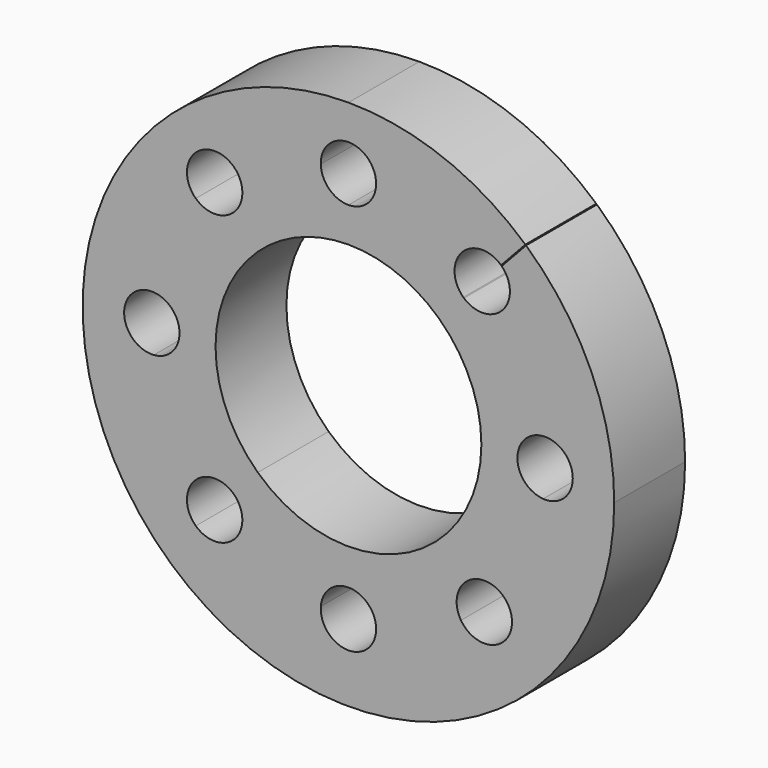
from build123d import *

# Parameters (mm, degrees)
F1_DEPTH = 25.4


# Not quite as in the source:
# - ends of sketch curves that miss each other by under 0.0002 mm in the source are joined


with BuildPart() as f1:
    # F0 (on Front) → F1 (new body)
    with BuildSketch(Plane.XZ):
        with BuildLine():
            ThreePointArc((7.9345325801, 55.8050164826), (5.535399088, 50.3331676174), (0, 48.0845394904))
            ThreePointArc((0, 48.0845394904), (-5.53484385, 50.3326274112), (-7.9344900677, 55.8034677281))
            ThreePointArc((-7.9344900677, 55.8034677281), (-20.6052011609, 52.4624086595), (-32.1621766165, 46.2861708383))
            ThreePointArc((-32.1621766165, 46.2861708383), (-30.8592654267, 43.9476457313), (-30.4078463876, 41.3089911317))
            ThreePointArc((-30.4078463876, 41.3089911317), (-31.0665806395, 38.1430038554), (-32.9334464969, 35.5025080461))
            ThreePointArc((-32.9334464969, 35.5025080461), (-38.3527879746, 33.37149462), (-43.7681241803, 35.5126658077))
            ThreePointArc((-43.7681241803, 35.5126658077), (-51.6631141521, 22.5336801806), (-55.8055284532, 7.9177526246))
            ThreePointArc((-55.8055284532, 7.9177526246), (-50.5579583584, 5.4112130729), (-48.4275815127, 0))
            ThreePointArc((-48.4275815127, 0), (-50.5584477046, -5.4117381745), (-55.8069604277, -7.917853693))
            ThreePointArc((-55.8069604277, -7.917853693), (-51.6665413057, -22.5360169357), (-43.772503534, -35.5174627239))
            ThreePointArc((-43.772503534, -35.5174627239), (-38.3573927277, -33.3769597298), (-32.9385406353, -35.5079735997))
            ThreePointArc((-32.9385406353, -35.5079735997), (-31.0716747779, -38.1484694089), (-30.412940526, -41.3144566852))
            ThreePointArc((-30.412940526, -41.3144566852), (-30.8645222652, -43.9535728332), (-32.1678845367, -46.2923987991))
            ThreePointArc((-32.1678845367, -46.2923987991), (-20.6005666804, -52.4744238707), (-7.9177489459, -55.8160418449))
            ThreePointArc((-7.9177489459, -55.8160418449), (0.0007699496, -48.4381469932), (7.917857362, -55.8175779229))
            ThreePointArc((7.917857362, -55.8175779229), (20.6543242596, -52.4575865986), (32.263311311, -46.2335565237))
            ThreePointArc((32.263311311, -46.2335565237), (31.0776824279, -40.9625014731), (33.540338967, -36.1536492228))
            ThreePointArc((33.540338967, -36.1536492228), (38.5262504819, -34.0340714863), (43.7106191867, -35.607044642))
            ThreePointArc((43.7106191867, -35.607044642), (51.6543788303, -22.5889167608), (55.8178964863, -7.917853693))
            ThreePointArc((55.8178964863, -7.917853693), (48.4385176038, -0.0007177684), (55.8164645119, 7.9177526246))
            ThreePointArc((55.8164645119, 7.9177526246), (51.6724507462, 22.537346487), (43.7740191713, 35.5188777315))
            ThreePointArc((43.7740191713, 35.5188777315), (38.4803716898, 33.3779972711), (33.1194704023, 35.3444179256))
            ThreePointArc((33.1194704023, 35.3444179256), (33.0283665185, 35.4254890622), (32.9385189369, 35.5079503192))
            ThreePointArc((32.9385189369, 35.5079503192), (30.4331832399, 40.7476116526), (32.166542765, 46.2907355552))
            ThreePointArc((32.166542765, 46.2907355552), (20.6072932493, 52.4658819521), (7.9345325801, 55.8050164826))
        make_face()
        with BuildLine():
            ThreePointArc((0, 38.1), (13.962710806, 35.4492976933), (25.9825875048, 27.8660213621))
            ThreePointArc((25.9825875048, 27.8660213621), (34.9475216227, 15.1899725896), (38.1109370587, -0.010193824))
            ThreePointArc((38.1109370587, -0.010193824), (15.1973926464, -34.9527404783), (-25.9825835021, -27.8660170726))
            ThreePointArc((-25.9825835021, -27.8660170726), (-38.1, 0), (-25.9825875048, 27.8660213621))
            ThreePointArc((-25.9825875048, 27.8660213621), (-13.962710806, 35.4492976933), (0, 38.1))
        make_face(mode=Mode.SUBTRACT)
        with BuildLine():
            ThreePointArc((-32.1621766165, 46.2861708383), (-20.6052011609, 52.4624086595), (-7.9344900677, 55.8034677281))
            ThreePointArc((-7.9344900677, 55.8034677281), (-5.6894120792, 61.5568833403), (0, 63.9595394904))
            Line((0, 63.9595394904), (0, 73.9440789808))
            ThreePointArc((0, 73.9440789808), (-27.1479472531, 68.9440014522), (-50.7331165271, 54.5999571944))
            Line((-50.7331165271, 54.5999571944), (-43.7572462783, 47.1154742172))
            ThreePointArc((-43.7572462783, 47.1154742172), (-37.7790864379, 49.2262669207), (-32.1621766165, 46.2861708383))
        make_face()
        with BuildLine():
            ThreePointArc((7.9375, 56.0220394904), (7.9367581103, 55.9135178434), (7.9345325801, 55.8050164826))
            ThreePointArc((7.9345325801, 55.8050164826), (20.6072932493, 52.4658819521), (32.166542765, 46.2907355552))
            ThreePointArc((32.166542765, 46.2907355552), (37.7835970754, 49.2316689925), (43.7623187183, 47.1209164903))
            Line((43.7623187183, 47.1209164903), (50.7331165271, 54.5999571944))
            ThreePointArc((50.7331165271, 54.5999571944), (27.1479472531, 68.9440014522), (0, 73.9440789808))
            Line((0, 73.9440789808), (0, 63.9595394904))
            ThreePointArc((0, 63.9595394904), (5.6126600757, 61.634699566), (7.9375, 56.0220394904))
        make_face()
        with BuildLine():
            ThreePointArc((-43.7681241803, 35.5126658077), (-46.2828428993, 41.3164327187), (-43.7572462783, 47.1154742172))
            Line((-43.7572462783, 47.1154742172), (-50.7331165271, 54.5999571944))
            ThreePointArc((-50.7331165271, 54.5999571944), (-31.1494504015, -71.7983666167), (76.2, -2.2559210192))
            ThreePointArc((76.2, -2.2559210192), (69.5922116943, 28.7821857449), (50.9148537664, 54.4372678657))
            Line((50.9148537664, 54.4372678657), (43.9381604406, 46.9519018008))
            ThreePointArc((43.9381604406, 46.9519018008), (45.6769666267, 44.3682185312), (46.2879188276, 41.3144334048))
            ThreePointArc((46.2879188276, 41.3144334048), (45.6323737155, 38.1557882425), (43.7740191713, 35.5188777315))
            ThreePointArc((43.7740191713, 35.5188777315), (51.6724507462, 22.537346487), (55.8164645119, 7.9177526246))
            ThreePointArc((55.8164645119, 7.9177526246), (61.7872306442, 5.8071231544), (64.3135175714, 0))
            ThreePointArc((64.3135175714, 0), (61.7877557458, -5.8066338081), (55.8178964863, -7.917853693))
            ThreePointArc((55.8178964863, -7.917853693), (51.6543788303, -22.5889167608), (43.7106191867, -35.607044642))
            ThreePointArc((43.7106191867, -35.607044642), (46.0506031098, -38.4080721744), (46.8897388577, -41.9601323083))
            ThreePointArc((46.8897388577, -41.9601323083), (46.2310046059, -45.1261195846), (44.3641387485, -47.7666153939))
            ThreePointArc((44.3641387485, -47.7666153939), (37.9546080225, -49.8346887381), (32.263311311, -46.2335565237))
            ThreePointArc((32.263311311, -46.2335565237), (20.6543242596, -52.4575865986), (7.917857362, -55.8175779229))
            ThreePointArc((7.917857362, -55.8175779229), (7.9325878205, -56.0964396499), (7.9375, -56.3756469558))
            ThreePointArc((7.9375, -56.3756469558), (-0.2799767777, -64.3082076555), (-7.9177489459, -55.8160418449))
            ThreePointArc((-7.9177489459, -55.8160418449), (-20.6005666804, -52.4744238707), (-32.1678845367, -46.2923987991))
            ThreePointArc((-32.1678845367, -46.2923987991), (-37.784668716, -49.2317673719), (-43.7623404168, -47.1209397708))
            ThreePointArc((-43.7623404168, -47.1209397708), (-46.2879374814, -41.3214088869), (-43.772503534, -35.5174627239))
            ThreePointArc((-43.772503534, -35.5174627239), (-51.6665413057, -22.5360169357), (-55.8069604277, -7.917853693))
            ThreePointArc((-55.8069604277, -7.917853693), (-64.3025814803, 0.0007177684), (-55.8055284532, 7.9177526246))
            ThreePointArc((-55.8055284532, 7.9177526246), (-51.6631141521, 22.5336801806), (-43.7681241803, 35.5126658077))
        make_face()
    extrude(amount=F1_DEPTH)


solid = f1.part
